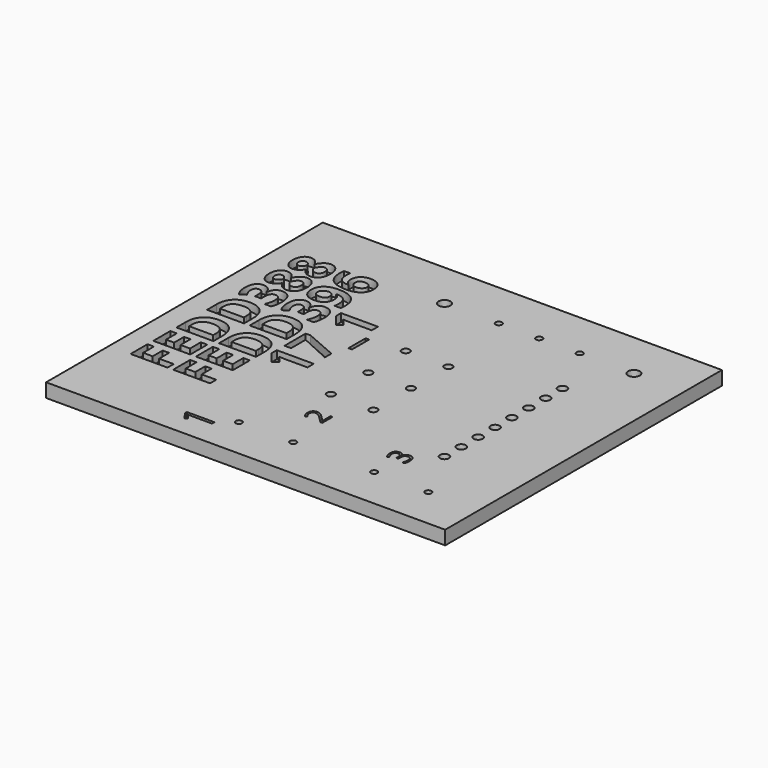
from build123d import *

# Parameters (mm, degrees)
F0_W           = 75
F0_H           = 65
F1_DEPTH       = 2.6
F2_TEXT_SIZE   = 9.7222222222
F2_TEXT_SIZE_2 = 7.24801812
F2_TEXT_SIZE_3 = 5.1460734388
F2_TEXT_SIZE_4 = 5.1905920519
F3_DEPTH       = 1.5
F4_R           = 0.85
F4_R_2         = 0.75
F4_R_3         = 0.6
F4_R_4         = 1.1
F5_DEPTH       = 2.6


# Not quite as in the source:
# - Text() gives the source's letters only with a copy of the font that has no kerning and outlines rounded to 1/6400 em; it was checked with that copy


with BuildPart() as f1:
    # F0 (on Top) → F1 (new body)
    with BuildSketch(Plane.XY):
        with Locations((-5.6587231159, 10.8350909071)):
            Rectangle(F0_W, F0_H)
    extrude(amount=F1_DEPTH)

    # F2 (on face) → F3 (cut)
    with BuildSketch(Plane.XY.offset(2.6)):
        with Locations(Location((-32.1587231159, -7.7649090929), (0, 0, 90))):
            Text('FEDD388', F2_TEXT_SIZE, font='Open Sans', font_style=FontStyle.BOLD, text_align=(TextAlign.LEFT, TextAlign.BOTTOM))
        with Locations(Location((-15.9401500695, -18.6649090929), (0, 0, 90))):
            Text('1', F2_TEXT_SIZE_2, font='Open Sans', text_align=(TextAlign.LEFT, TextAlign.BOTTOM))
        with Locations(Location((-3.45355024, -6.6649090929), (0, 0, 90))):
            Text('2', F2_TEXT_SIZE_3, font='Open Sans', text_align=(TextAlign.LEFT, TextAlign.BOTTOM))
        with Locations(Location((14.0877261274, -9.1649090929), (0, 0, 90))):
            Text('3', F2_TEXT_SIZE_4, font='Open Sans', text_align=(TextAlign.LEFT, TextAlign.BOTTOM))
        with Locations(Location((-24.1587231159, -7.7649090929), (0, 0, 90))):
            Text('FEDD396', F2_TEXT_SIZE, font='Open Sans', font_style=FontStyle.BOLD, text_align=(TextAlign.LEFT, TextAlign.BOTTOM))
        with Locations(Location((-16.1587231159, 3.4369138237), (0, 0, 90))):
            Text('17_1', F2_TEXT_SIZE, font='Open Sans', font_style=FontStyle.BOLD, text_align=(TextAlign.LEFT, TextAlign.BOTTOM))
    extrude(amount=-F3_DEPTH, mode=Mode.SUBTRACT)

    # F4 (on face) → F5 (cut, through all)
    with BuildSketch(Plane.XY.offset(2.6)):
        with Locations((17.2412768841, -3.5849090929)):
            Circle(F4_R)
        with Locations((17.2412768841, 0.3750909071)):
            Circle(F4_R)
        with Locations((17.2412768841, 4.3350909071)):
            Circle(F4_R)
        with Locations((17.2412768841, 8.2950909071)):
            Circle(F4_R)
        with Locations((17.2412768841, 12.2550909071)):
            Circle(F4_R)
        with Locations((17.2412768841, 16.2150909071)):
            Circle(F4_R)
        with Locations((17.2412768841, 20.1750909071)):
            Circle(F4_R)
        with Locations((17.2412768841, 24.1350909071)):
            Circle(F4_R)
        with Locations((-8.1587231159, 1.4750909071)):
            Circle(F4_R_2)
        with Locations((-8.1587231159, 10.2750909071)):
            Circle(F4_R_2)
        with Locations((-8.1587231159, 19.0750909071)):
            Circle(F4_R_2)
        with Locations((-0.1587231159, 1.4750909071)):
            Circle(F4_R_2)
        with Locations((-0.1587231159, 10.2750909071)):
            Circle(F4_R_2)
        with Locations((-0.1587231159, 19.0750909071)):
            Circle(F4_R_2)
        with Locations((-13.1587231159, -13.8749090929)):
            Circle(F4_R_3)
        with Locations((-13.1587231159, 34.4250909071)):
            Circle(F4_R_4)
        with Locations((22.4412768841, 34.4250909071)):
            Circle(F4_R_4)
        with Locations((22.4412768841, -13.8749090929)):
            Circle(F4_R_3)
        with Locations((-2.9587231159, 34.4250909071)):
            Circle(F4_R_3)
        with Locations((4.6412768841, 34.4250909071)):
            Circle(F4_R_3)
        with Locations((12.2412768841, 34.4250909071)):
            Circle(F4_R_3)
        with Locations((-2.9587231159, -13.8749090929)):
            Circle(F4_R_3)
        with Locations((12.2412768841, -13.8749090929)):
            Circle(F4_R_3)
    extrude(amount=-F5_DEPTH, mode=Mode.SUBTRACT)


solid = f1.part
